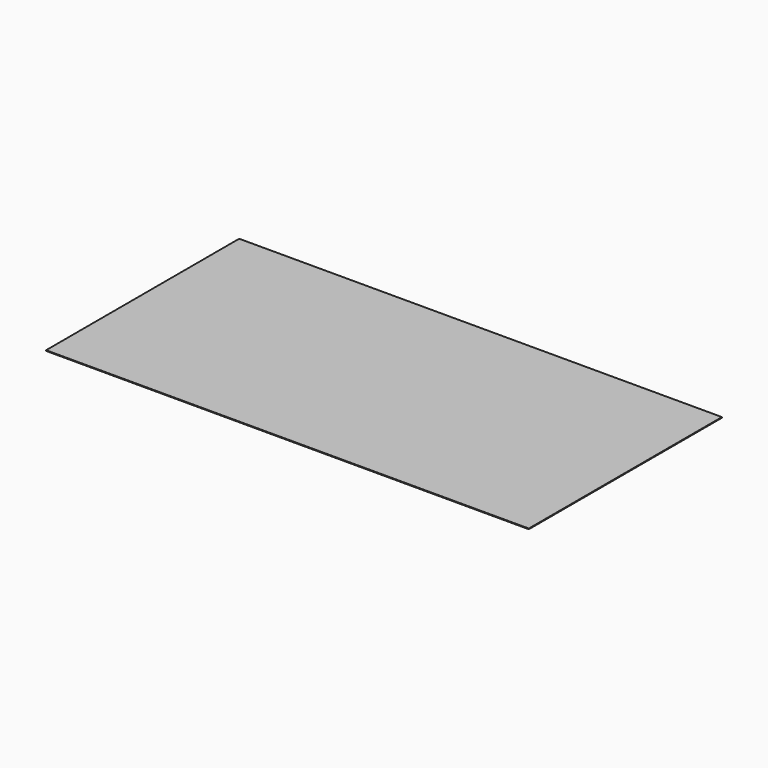
from build123d import *

# Parameters (mm, degrees)
F0_W     = 3962.4
F0_H     = 4572
F0_W_2   = 3048
F0_H_2   = 1828.8
F4_DEPTH = 25.4


# Not quite as in the source:
# - the program builds the solid bodies; features that only make, move or delete a surface that nothing else refers to are left out


with BuildPart() as f4:
    # F0 (on Top) → F4 (new body)
    with BuildSketch(Plane.XY):
        Polygon((4876.8, 914.4), (4876.8, 4572), (-3048, 4572), (-3048, 0), (-3048, -1828.8), (-5181.6, -1828.8), (-5181.6, -4572), (4876.8, -4572), (4876.8, -914.4), (6096, -914.4), (6096, 914.4), align=None)
        with Locations((-5029.2, 2286)):
            Rectangle(F0_W, F0_H)
        Polygon((-3048, -1828.8), (-3048, 0), (-7010.4, 0), (-7010.4, -1828.8), (-5181.6, -1828.8), align=None)
        Polygon((-7010.4, 0), (-7010.4, 4572), (-9144, 4572), (-9144, -1828.8), (-7010.4, -1828.8), align=None)
        Polygon((-7010.4, -1828.8), (-9144, -1828.8), (-9144, -4572), (-5181.6, -4572), (-5181.6, -1828.8), align=None)
        Polygon((9144, 914.4), (9144, 4572), (4876.8, 4572), (4876.8, 914.4), (6096, 914.4), align=None)
        with Locations((7620, 0)):
            Rectangle(F0_W_2, F0_H_2)
        Polygon((9144, -4572), (9144, -914.4), (6096, -914.4), (4876.8, -914.4), (4876.8, -4572), align=None)
    extrude(amount=F4_DEPTH)


solid = f4.part
